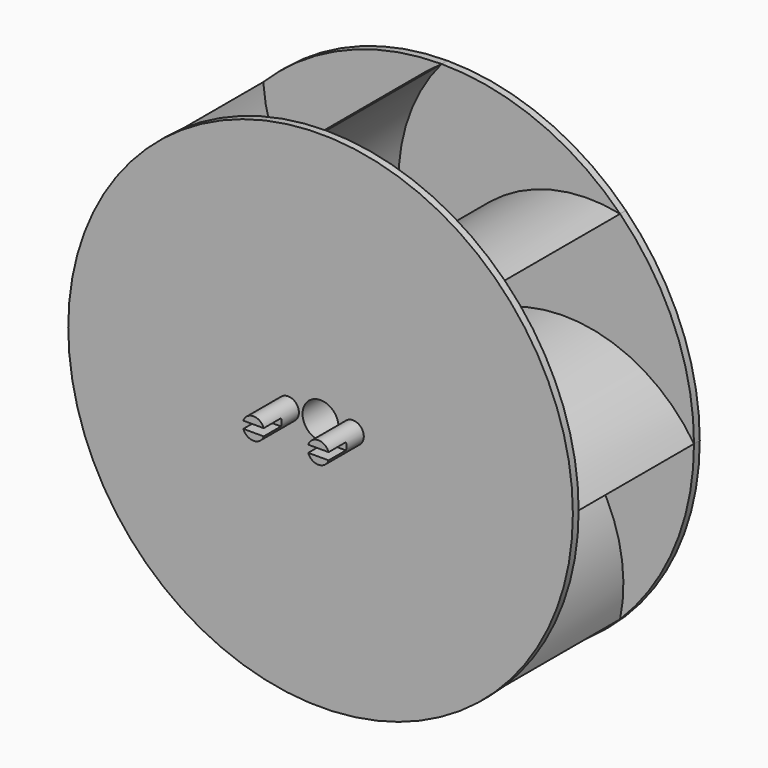
from build123d import *

# Parameters (mm, degrees)
F0_R     = 2.5
F1_DEPTH = 20
F2_DEPTH = 1
F3_R     = 35
F3_R_2   = 1.5
F3_R_3   = 2.5
F4_DEPTH = 1
F5_DEPTH = 7
F8_DEPTH = 3


with BuildPart() as f1:
    # F0 (on Front) → F1 (new body)
    with BuildSketch(Plane.XZ):
        with BuildLine():
            ThreePointArc((5.5655123118, 2.2416673945), (20.6488442828, 5.9277985889), (35, 0))
            ThreePointArc((35, 0), (20.2866870884, 9.5155994681), (3.3649940235, 4.9675763931))
            ThreePointArc((3.3649940235, 4.9675763931), (2.8709960308, 5.2685274784), (2.3503132806, 5.5205097122))
            ThreePointArc((2.3503132806, 5.5205097122), (10.4093512363, 18.7925243957), (24.7487373415, 24.7487373415))
            ThreePointArc((24.7487373415, 24.7487373415), (7.6163090971, 21.073398919), (-1.133196861, 5.8920170463))
            ThreePointArc((-1.133196861, 5.8920170463), (-1.6953107447, 5.755512269), (-2.2416673945, 5.5655123118))
            ThreePointArc((-2.2416673945, 5.5655123118), (-5.9277985889, 20.6488442828), (0, 35))
            ThreePointArc((0, 35), (-9.5155994681, 20.2866870884), (-4.9675763931, 3.3649940235))
            ThreePointArc((-4.9675763931, 3.3649940235), (-5.2685274784, 2.8709960308), (-5.5205097122, 2.3503132806))
            ThreePointArc((-5.5205097122, 2.3503132806), (-18.7925243957, 10.4093512363), (-24.7487373415, 24.7487373415))
            ThreePointArc((-24.7487373415, 24.7487373415), (-21.073398919, 7.6163090971), (-5.8920170463, -1.133196861))
            ThreePointArc((-5.8920170463, -1.133196861), (-5.755512269, -1.6953107447), (-5.5655123118, -2.2416673945))
            ThreePointArc((-5.5655123118, -2.2416673945), (-20.6488442828, -5.9277985889), (-35, 0))
            ThreePointArc((-35, 0), (-20.2866870884, -9.5155994681), (-3.3649940235, -4.9675763931))
            ThreePointArc((-3.3649940235, -4.9675763931), (-2.8709960308, -5.2685274784), (-2.3503132806, -5.5205097122))
            ThreePointArc((-2.3503132806, -5.5205097122), (-10.4093512363, -18.7925243957), (-24.7487373415, -24.7487373415))
            ThreePointArc((-24.7487373415, -24.7487373415), (-7.6163090971, -21.073398919), (1.133196861, -5.8920170463))
            ThreePointArc((1.133196861, -5.8920170463), (1.6953107447, -5.755512269), (2.2416673945, -5.5655123118))
            ThreePointArc((2.2416673945, -5.5655123118), (5.9277985889, -20.6488442828), (0, -35))
            ThreePointArc((0, -35), (9.5155994681, -20.2866870884), (4.9675763931, -3.3649940235))
            ThreePointArc((4.9675763931, -3.3649940235), (5.2685274784, -2.8709960308), (5.5205097122, -2.3503132806))
            ThreePointArc((5.5205097122, -2.3503132806), (18.7925243957, -10.4093512363), (24.7487373415, -24.7487373415))
            ThreePointArc((24.7487373415, -24.7487373415), (21.073398919, -7.6163090971), (5.8920170463, 1.133196861))
            ThreePointArc((5.8920170463, 1.133196861), (5.755512269, 1.6953107447), (5.5655123118, 2.2416673945))
        make_face()
        Circle(F0_R, mode=Mode.SUBTRACT)
    extrude(amount=F1_DEPTH)

    # F0 (on Front) → F2 (join)
    with BuildSketch(Plane.XZ):
        with BuildLine():
            ThreePointArc((3.3649940235, 4.9675763931), (20.2866870884, 9.5155994681), (35, 0))
            ThreePointArc((35, 0), (32.3357836379, 13.3939201328), (24.7487373415, 24.7487373415))
            ThreePointArc((24.7487373415, 24.7487373415), (10.4093512363, 18.7925243957), (2.3503132806, 5.5205097122))
            ThreePointArc((2.3503132806, 5.5205097122), (2.8709960308, 5.2685274784), (3.3649940235, 4.9675763931))
        make_face()
        with BuildLine():
            ThreePointArc((5.5655123118, 2.2416673945), (20.6488442828, 5.9277985889), (35, 0))
            ThreePointArc((35, 0), (20.2866870884, 9.5155994681), (3.3649940235, 4.9675763931))
            ThreePointArc((3.3649940235, 4.9675763931), (2.8709960308, 5.2685274784), (2.3503132806, 5.5205097122))
            ThreePointArc((2.3503132806, 5.5205097122), (10.4093512363, 18.7925243957), (24.7487373415, 24.7487373415))
            ThreePointArc((24.7487373415, 24.7487373415), (7.6163090971, 21.073398919), (-1.133196861, 5.8920170463))
            ThreePointArc((-1.133196861, 5.8920170463), (-1.6953107447, 5.755512269), (-2.2416673945, 5.5655123118))
            ThreePointArc((-2.2416673945, 5.5655123118), (-5.9277985889, 20.6488442828), (0, 35))
            ThreePointArc((0, 35), (-9.5155994681, 20.2866870884), (-4.9675763931, 3.3649940235))
            ThreePointArc((-4.9675763931, 3.3649940235), (-5.2685274784, 2.8709960308), (-5.5205097122, 2.3503132806))
            ThreePointArc((-5.5205097122, 2.3503132806), (-18.7925243957, 10.4093512363), (-24.7487373415, 24.7487373415))
            ThreePointArc((-24.7487373415, 24.7487373415), (-21.073398919, 7.6163090971), (-5.8920170463, -1.133196861))
            ThreePointArc((-5.8920170463, -1.133196861), (-5.755512269, -1.6953107447), (-5.5655123118, -2.2416673945))
            ThreePointArc((-5.5655123118, -2.2416673945), (-20.6488442828, -5.9277985889), (-35, 0))
            ThreePointArc((-35, 0), (-20.2866870884, -9.5155994681), (-3.3649940235, -4.9675763931))
            ThreePointArc((-3.3649940235, -4.9675763931), (-2.8709960308, -5.2685274784), (-2.3503132806, -5.5205097122))
            ThreePointArc((-2.3503132806, -5.5205097122), (-10.4093512363, -18.7925243957), (-24.7487373415, -24.7487373415))
            ThreePointArc((-24.7487373415, -24.7487373415), (-7.6163090971, -21.073398919), (1.133196861, -5.8920170463))
            ThreePointArc((1.133196861, -5.8920170463), (1.6953107447, -5.755512269), (2.2416673945, -5.5655123118))
            ThreePointArc((2.2416673945, -5.5655123118), (5.9277985889, -20.6488442828), (0, -35))
            ThreePointArc((0, -35), (9.5155994681, -20.2866870884), (4.9675763931, -3.3649940235))
            ThreePointArc((4.9675763931, -3.3649940235), (5.2685274784, -2.8709960308), (5.5205097122, -2.3503132806))
            ThreePointArc((5.5205097122, -2.3503132806), (18.7925243957, -10.4093512363), (24.7487373415, -24.7487373415))
            ThreePointArc((24.7487373415, -24.7487373415), (21.073398919, -7.6163090971), (5.8920170463, 1.133196861))
            ThreePointArc((5.8920170463, 1.133196861), (5.755512269, 1.6953107447), (5.5655123118, 2.2416673945))
        make_face()
        Circle(F0_R, mode=Mode.SUBTRACT)
        with BuildLine():
            ThreePointArc((24.7487373415, -24.7487373415), (32.3357836379, -13.3939201328), (35, 0))
            ThreePointArc((35, 0), (20.6488442828, 5.9277985889), (5.5655123118, 2.2416673945))
            ThreePointArc((5.5655123118, 2.2416673945), (5.755512269, 1.6953107447), (5.8920170463, 1.133196861))
            ThreePointArc((5.8920170463, 1.133196861), (21.073398919, -7.6163090971), (24.7487373415, -24.7487373415))
        make_face()
        with BuildLine():
            ThreePointArc((-1.133196861, 5.8920170463), (7.6163090971, 21.073398919), (24.7487373415, 24.7487373415))
            ThreePointArc((24.7487373415, 24.7487373415), (13.3939201328, 32.3357836379), (0, 35))
            ThreePointArc((0, 35), (-5.9277985889, 20.6488442828), (-2.2416673945, 5.5655123118))
            ThreePointArc((-2.2416673945, 5.5655123118), (-1.6953107447, 5.755512269), (-1.133196861, 5.8920170463))
        make_face()
        with BuildLine():
            ThreePointArc((0, -35), (13.3939201328, -32.3357836379), (24.7487373415, -24.7487373415))
            ThreePointArc((24.7487373415, -24.7487373415), (18.7925243957, -10.4093512363), (5.5205097122, -2.3503132806))
            ThreePointArc((5.5205097122, -2.3503132806), (5.2685274784, -2.8709960308), (4.9675763931, -3.3649940235))
            ThreePointArc((4.9675763931, -3.3649940235), (9.5155994681, -20.2866870884), (0, -35))
        make_face()
        with BuildLine():
            ThreePointArc((-4.9675763931, 3.3649940235), (-9.5155994681, 20.2866870884), (0, 35))
            ThreePointArc((0, 35), (-13.3939201328, 32.3357836379), (-24.7487373415, 24.7487373415))
            ThreePointArc((-24.7487373415, 24.7487373415), (-18.7925243957, 10.4093512363), (-5.5205097122, 2.3503132806))
            ThreePointArc((-5.5205097122, 2.3503132806), (-5.2685274784, 2.8709960308), (-4.9675763931, 3.3649940235))
        make_face()
        with BuildLine():
            ThreePointArc((-24.7487373415, -24.7487373415), (-13.3939201328, -32.3357836379), (0, -35))
            ThreePointArc((0, -35), (5.9277985889, -20.6488442828), (2.2416673945, -5.5655123118))
            ThreePointArc((2.2416673945, -5.5655123118), (1.6953107447, -5.755512269), (1.133196861, -5.8920170463))
            ThreePointArc((1.133196861, -5.8920170463), (-7.6163090971, -21.073398919), (-24.7487373415, -24.7487373415))
        make_face()
        with BuildLine():
            ThreePointArc((-5.8920170463, -1.133196861), (-21.073398919, 7.6163090971), (-24.7487373415, 24.7487373415))
            ThreePointArc((-24.7487373415, 24.7487373415), (-32.3357836379, 13.3939201328), (-35, 0))
            ThreePointArc((-35, 0), (-20.6488442828, -5.9277985889), (-5.5655123118, -2.2416673945))
            ThreePointArc((-5.5655123118, -2.2416673945), (-5.755512269, -1.6953107447), (-5.8920170463, -1.133196861))
        make_face()
        with BuildLine():
            ThreePointArc((-35, 0), (-32.3357836379, -13.3939201328), (-24.7487373415, -24.7487373415))
            ThreePointArc((-24.7487373415, -24.7487373415), (-10.4093512363, -18.7925243957), (-2.3503132806, -5.5205097122))
            ThreePointArc((-2.3503132806, -5.5205097122), (-2.8709960308, -5.2685274784), (-3.3649940235, -4.9675763931))
            ThreePointArc((-3.3649940235, -4.9675763931), (-20.2866870884, -9.5155994681), (-35, 0))
        make_face()
    extrude(amount=-F2_DEPTH)

    # F3 (on face) → F4 (join)
    with BuildSketch(Plane.XZ.offset(20)):
        Circle(F3_R)
        with Locations((-4.5, 0)):
            Circle(F3_R_2, mode=Mode.SUBTRACT)
        Circle(F3_R_3, mode=Mode.SUBTRACT)
        with Locations((4.5, 0)):
            Circle(F3_R_2, mode=Mode.SUBTRACT)
    extrude(amount=F4_DEPTH)

    # F5 (add): faces of the model
    f5_faces = [f1.faces().sort_by_distance(p)[0] for p in [
        (4.5, -20, 0),
        (-4.5, -20, 0),
    ]]
    extrude(f5_faces, amount=F5_DEPTH)

    # F6 (on face) + F7 (on face) → F8 (cut)
    with BuildSketch(Plane.XZ.offset(27)):
        with BuildLine():
            Line((-3.0857864376, 0.5), (-5.9142135624, 0.5))
            ThreePointArc((-5.9142135624, 0.5), (-5.9783978395, 0.2536529681), (-6, 0))
            ThreePointArc((-6, 0), (-5.9783978395, -0.2536529681), (-5.9142135624, -0.5))
            Line((-5.9142135624, -0.5), (-3.0857864376, -0.5))
            ThreePointArc((-3.0857864376, -0.5), (-3.0216021605, -0.2536529681), (-3, 0))
            ThreePointArc((-3, 0), (-3.0216021605, 0.2536529681), (-3.0857864376, 0.5))
        make_face()
        with BuildLine():
            Line((-3, 0.5), (-3.0857864376, 0.5))
            ThreePointArc((-3.0857864376, 0.5), (-3.0216021605, 0.2536529681), (-3, 0))
            Line((-3, 0), (-3, 0.5))
        make_face()
    with BuildSketch(Plane.XZ.offset(27)):
        with BuildLine():
            Line((5.9142135624, 0.5), (3.0857864376, 0.5))
            ThreePointArc((3.0857864376, 0.5), (3.0216021605, 0.2536529681), (3, 0))
            ThreePointArc((3, 0), (3.0216021605, -0.2536529681), (3.0857864376, -0.5))
            Line((3.0857864376, -0.5), (5.9142135624, -0.5))
            ThreePointArc((5.9142135624, -0.5), (5.9783978395, -0.2536529681), (6, 0))
            ThreePointArc((6, 0), (5.9783978395, 0.2536529681), (5.9142135624, 0.5))
        make_face()
        with BuildLine():
            Line((6, 0.5), (5.9142135624, 0.5))
            ThreePointArc((5.9142135624, 0.5), (5.9783978395, 0.2536529681), (6, 0))
            Line((6, 0), (6, 0.5))
        make_face()
    extrude(amount=-F8_DEPTH, mode=Mode.SUBTRACT)


solid = f1.part
